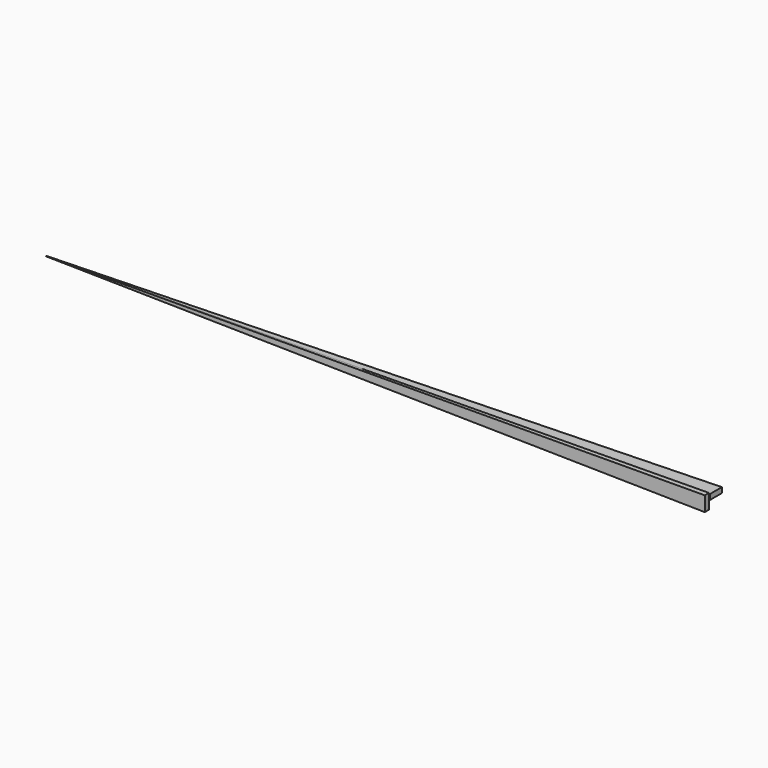
from build123d import *

# Parameters (mm, degrees)
F0_W      = 32
F0_H      = 90
F1_DEPTH  = 4000
F3_DEPTH  = 32.001
F5_DEPTH  = 89.9993800437
F6_DEPTH  = 0.3969928722
F7_W      = 90
F7_H      = 32
F7_W_2    = 45
F8_DEPTH  = 4000
F10_DEPTH = 81.001
F12_DEPTH = 125.99589731


with BuildPart() as f1:
    # F0 (on Right) → F1 (new body)
    with BuildSketch(Plane.YZ):
        with Locations((11, -20)):
            Rectangle(F0_W, F0_H)
    extrude(amount=F1_DEPTH)

    # F2 (on face) → F3 (cut, through all)
    with BuildSketch(Plane.XZ.offset(5)):
        Polygon((0, 25), (0, 1), (4000, 25), align=None)
        Polygon((4000, -65), (0, -1), (0, -65), align=None)
    extrude(amount=-F3_DEPTH, mode=Mode.SUBTRACT)

    # F4 (on face) → F5 (cut, through all)
    with BuildSketch(Plane(origin=(-0.005999784, 0, 0.9999640013), x_dir=(0.9999820005, 0, 0.005999892), z_dir=(-0.005999892, 0, 0.9999820005))):
        Polygon((0.005999892, 27), (0.005999892, 0.9999820005), (4000.077999244, 27), align=None)
        Polygon((4000.077999244, -5), (0.005999892, -0.9999820005), (0.005999892, -5), align=None)
    extrude(amount=-F5_DEPTH, mode=Mode.SUBTRACT)

    # F6 (cut, through all): faces of the model
    f6_faces = [f1.faces().sort_by_distance(p)[0] for p in [
        (0.0060005761, -2.9999910002, -9.60092e-05),
        (0.0060005761, 13.9999910002, -9.60092e-05),
    ]]
    extrude(f6_faces, amount=-F6_DEPTH, mode=Mode.SUBTRACT)


with BuildPart() as f8:
    # F7 (on Right) → F8 (new body)
    with BuildSketch(Plane.YZ):
        with Locations((80, 0)):
            Rectangle(F7_W, F7_H)
        with Locations((12.5, 0)):
            Rectangle(F7_W_2, F7_H)
    extrude(amount=F8_DEPTH)

    # F9 (on face) → F10 (cut, through all)
    with BuildSketch(Plane.XY.offset(16)):
        Polygon((4000, 35), (0, -1), (0, -10), (4000, -10), align=None)
        Polygon((0, 125), (0, 1), (4000, 125), align=None)
    extrude(amount=-F10_DEPTH, mode=Mode.SUBTRACT)

    # F11 (on face) → F12 (cut, through all)
    with BuildSketch(Plane(origin=(0.0089992711, -0.9999190066, 0), x_dir=(0.9999595025, 0.0089996355, 0), z_dir=(0.0089996355, -0.9999595025, 0))):
        Polygon((-0.0089996355, 16), (-0.0089996355, 1), (4000.1529970841, 16), align=None)
        Polygon((4000.1529970841, -16), (-0.0089996355, -1), (-0.0089996355, -16), align=None)
    extrude(amount=-F12_DEPTH, mode=Mode.SUBTRACT)


solid = Compound([f1.part, f8.part])
